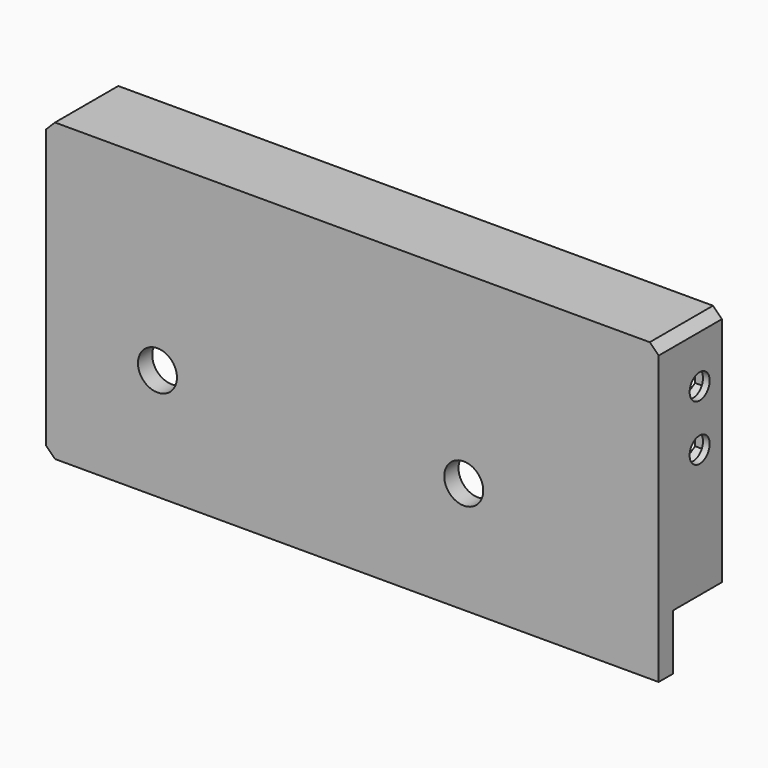
from build123d import *

# Parameters (mm, degrees)
F0_W      = 110
F0_H      = 50
F0_R      = 3.5
F1_DEPTH  = 3.2
F2_W      = 3.2
F2_H      = 40
F3_DEPTH  = 14.2
F4_R      = 2.25
F5_DEPTH  = 110.001
F6_W      = 110
F6_H      = 3.2
F7_DEPTH  = 14.2
F8_SIZE   = 1.6
F10_DEPTH = 2


# Not quite as in the source:
# - a pattern or mirror of a feature is missing from the dataset's text; its kind, count and spacing are read off the source's solid


with BuildPart() as f1:
    # F0 (on Front) → F1 (new body)
    with BuildSketch(Plane.XZ):
        Rectangle(F0_W, F0_H)
        with Locations((-35, -5)):
            Circle(F0_R, mode=Mode.SUBTRACT)
        with Locations((20, -5)):
            Circle(F0_R, mode=Mode.SUBTRACT)
    extrude(amount=F1_DEPTH)

    # F2 (on face) → F3 (join)
    with BuildSketch(Plane.XZ.offset(3.2)):
        with Locations((53.4, 5)):
            Rectangle(F2_W, F2_H)
        with Locations((-53.4, 5)):
            Rectangle(F2_W, F2_H)
    extrude(amount=-F3_DEPTH)

    # F4 (on face) → F5 (cut, through all)
    with BuildSketch(Plane.YZ.offset(55)):
        with Locations((6, 18)):
            Circle(F4_R)
        with Locations((6, 8)):
            Circle(F4_R)
    extrude(amount=-F5_DEPTH, mode=Mode.SUBTRACT)

    # F6 (on face) → F7 (join)
    with BuildSketch(Plane.XZ.offset(3.2)):
        with Locations((0, 26.6)):
            Rectangle(F6_W, F6_H)
    extrude(amount=-F7_DEPTH)

    # F8
    f8_edges = [f1.edges().sort_by_distance(p)[0] for p in [
        (55, 3.9, 28.2),
        (-55, 3.9, 28.2),
        (-55, -1.6, -25),
    ]]
    chamfer(f8_edges, length=F8_SIZE)

    # F9 (on face) → F10 (cut)
    with BuildSketch(Plane(origin=(51.8, 0, 0), x_dir=(0, -1, 0), z_dir=(-1, 0, 0))):
        Polygon((-8.975, 9.7176170508), (-8.975, 6.2823829492), (-6, 4.5647658983), (-3.025, 6.2823829492), (-3.025, 9.7176170508), (-6, 11.4352341017), align=None)
        Polygon((-8.975, 19.7176170508), (-8.975, 16.2823829492), (-6, 14.5647658983), (-3.025, 16.2823829492), (-3.025, 19.7176170508), (-6, 21.4352341017), align=None)
    f10 = extrude(amount=-F10_DEPTH, mode=Mode.SUBTRACT)

    # F10_copies: F10 across plane
    add(f10.mirror(Plane(origin=(0, 0, 0), x_dir=(0, 0, -1), z_dir=(-1, 0, 0))), mode=Mode.SUBTRACT)


solid = f1.part
